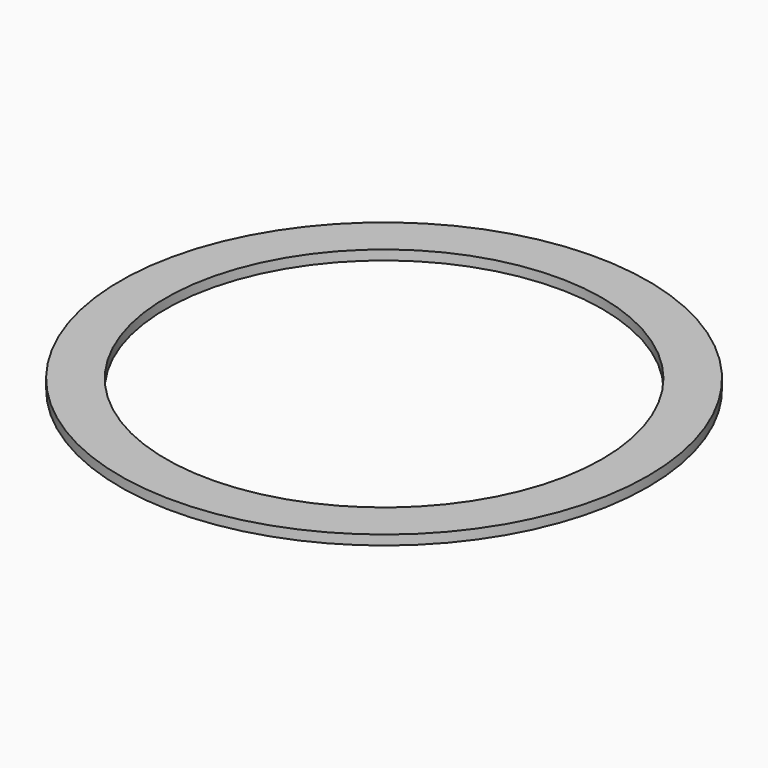
from build123d import *

# Parameters (mm, degrees)
F1_R     = 27.2213151776
F1_R_2   = 22.5
F2_DEPTH = 22
F3_DEPTH = 21


# Not quite as in the source:
# - the program builds the solid bodies; features that only make, move or delete a surface that nothing else refers to are left out


with BuildPart() as f2:
    # F1 (on Top) → F2 (new body)
    with BuildSketch(Plane.XY):
        Circle(F1_R)
        Circle(F1_R_2, mode=Mode.SUBTRACT)
    extrude(amount=-F2_DEPTH)

    # F3 (cut): a face of the model
    f3_faces = [f2.faces().sort_by_distance(p)[0] for p in [
        (-26.4513801154, 0, 0),
    ]]
    extrude(f3_faces, amount=-F3_DEPTH, mode=Mode.SUBTRACT)


solid = f2.part
